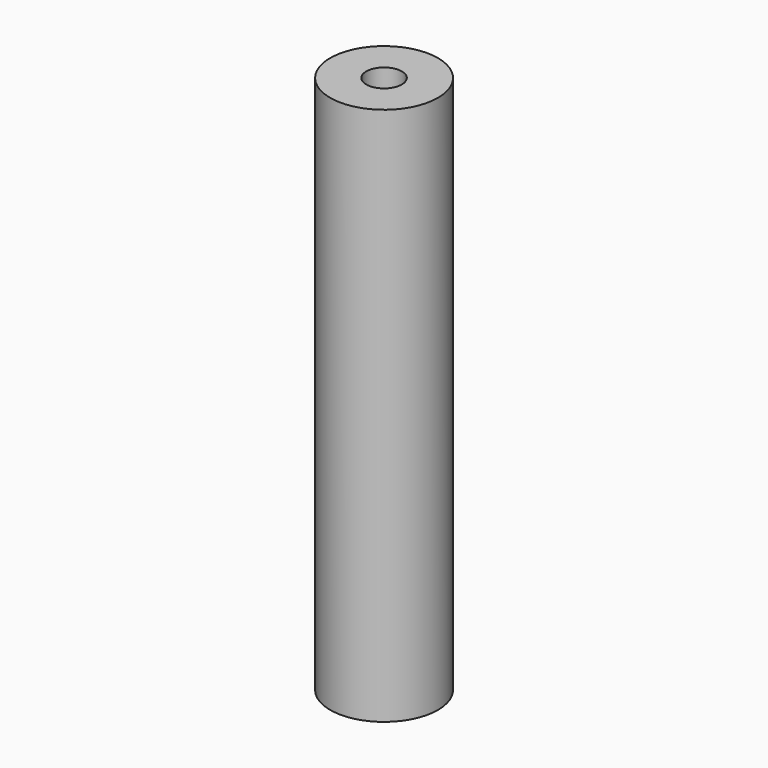
from build123d import *

# Parameters (mm, degrees)
F0_R     = 5.08
F0_R_2   = 1.6764
F1_DEPTH = 50.8


# Not quite as in the source:
# - a feature names something its author has since deleted; it is built from what else it names


with BuildPart() as f1:
    # F0 (on Top) → F1 (new body)
    with BuildSketch(Plane.XY):
        Circle(F0_R)
        Circle(F0_R_2, mode=Mode.SUBTRACT)
    extrude(amount=F1_DEPTH)


solid = f1.part
